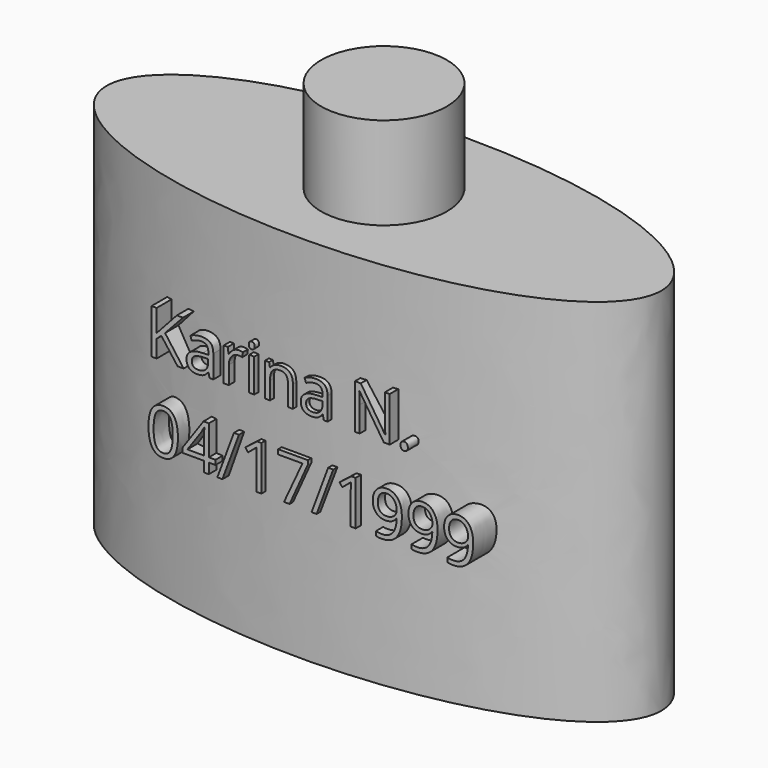
from build123d import *

# Parameters (mm, degrees)
F1_DEPTH     = 25.4
F2_R         = 4.3170881458
F3_DEPTH     = 6.35
F4_TEXT_SIZE = 4.2856800266
F5_DEPTH     = 7.62


# Not quite as in the source:
# - Text() gives the source's letters only with a copy of the font that has no kerning and outlines rounded to 1/6400 em; it was checked with that copy


with BuildPart() as f1:
    # F0 (on Top) → F1 (new body)
    with BuildSketch(Plane.XY):
        with BuildLine():
            add(Edge.make_bspline(
                [(19.05, 0), (19.05, 12.6902184546), (-9.525, 6.3451092273), (-38.1, 0), (-9.525, -6.3451092273), (19.05, -12.6902184546), (19.05, 0)],
                knots=[0, 0, 0, 2.0943951024, 2.0943951024, 4.1887902048, 4.1887902048, 6.2831853072, 6.2831853072, 6.2831853072], degree=2, weights=[1, 0.5, 1, 0.5, 1, 0.5, 1]))
        make_face()
    extrude(amount=F1_DEPTH)

    # F2 (on face) → F3 (join)
    with BuildSketch(Plane.XY.offset(25.4)):
        Circle(F2_R)
    extrude(amount=F3_DEPTH)

    # F4 (on Front) → F5 (join)
    with BuildSketch(Plane.XZ):
        with Locations((-10.2953286842, 15.1050845161)):
            Text('Karina N.', F4_TEXT_SIZE, font='Open Sans', text_align=(TextAlign.LEFT, TextAlign.BOTTOM))
        with Locations((-10.2953286842, 9.2765596799)):
            Text('04/17/1999', F4_TEXT_SIZE, font='Open Sans', text_align=(TextAlign.LEFT, TextAlign.BOTTOM))
    extrude(amount=F5_DEPTH)


solid = f1.part
